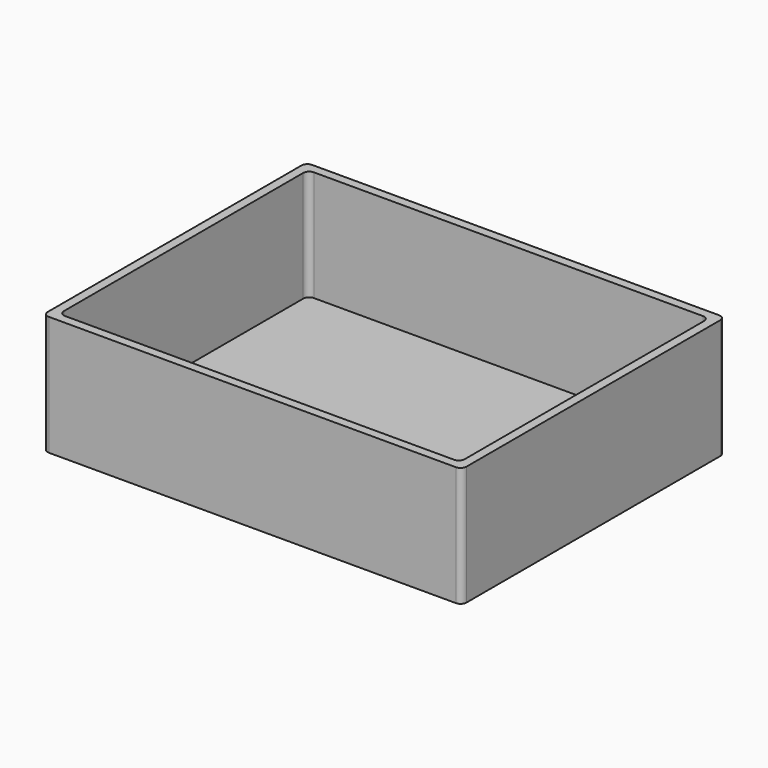
from build123d import *

# Parameters (mm, degrees)
F0_W     = 70
F0_H     = 55
F1_DEPTH = 20
F2_T     = -1.5
F3_R     = 1
F4_R     = 1
F5_R     = 1
F6_R     = 1
F7_R     = 1
F8_R     = 1
F9_R     = 1


with BuildPart() as f1:
    # F0 (on Top) → F1 (new body)
    with BuildSketch(Plane.XY):
        with Locations((35, 27.5)):
            Rectangle(F0_W, F0_H)
    extrude(amount=F1_DEPTH)

    # F2
    f2_openings = [f1.faces().sort_by_distance(p)[0] for p in [
        (35, 27.5, 20),
    ]]
    offset(amount=F2_T, openings=f2_openings)

    # F3
    f3_edges = [f1.edges().sort_by_distance(p)[0] for p in [
        (0, 55, 10),
        (1.5, 53.5, 10.75),
    ]]
    fillet(f3_edges, radius=F3_R)

    # F4
    f4_edges = [f1.edges().sort_by_distance(p)[0] for p in [
        (0, 0, 10),
    ]]
    fillet(f4_edges, radius=F4_R)

    # F5
    f5_edges = [f1.edges().sort_by_distance(p)[0] for p in [
        (70, 0, 10),
    ]]
    fillet(f5_edges, radius=F5_R)

    # F6
    f6_edges = [f1.edges().sort_by_distance(p)[0] for p in [
        (70, 55, 10),
    ]]
    fillet(f6_edges, radius=F6_R)

    # F7
    f7_edges = [f1.edges().sort_by_distance(p)[0] for p in [
        (68.5, 1.5, 10.75),
    ]]
    fillet(f7_edges, radius=F7_R)

    # F8
    f8_edges = [f1.edges().sort_by_distance(p)[0] for p in [
        (1.5, 1.5, 10.75),
    ]]
    fillet(f8_edges, radius=F8_R)

    # F9
    f9_edges = [f1.edges().sort_by_distance(p)[0] for p in [
        (68.5, 53.5, 10.75),
    ]]
    fillet(f9_edges, radius=F9_R)


solid = f1.part
